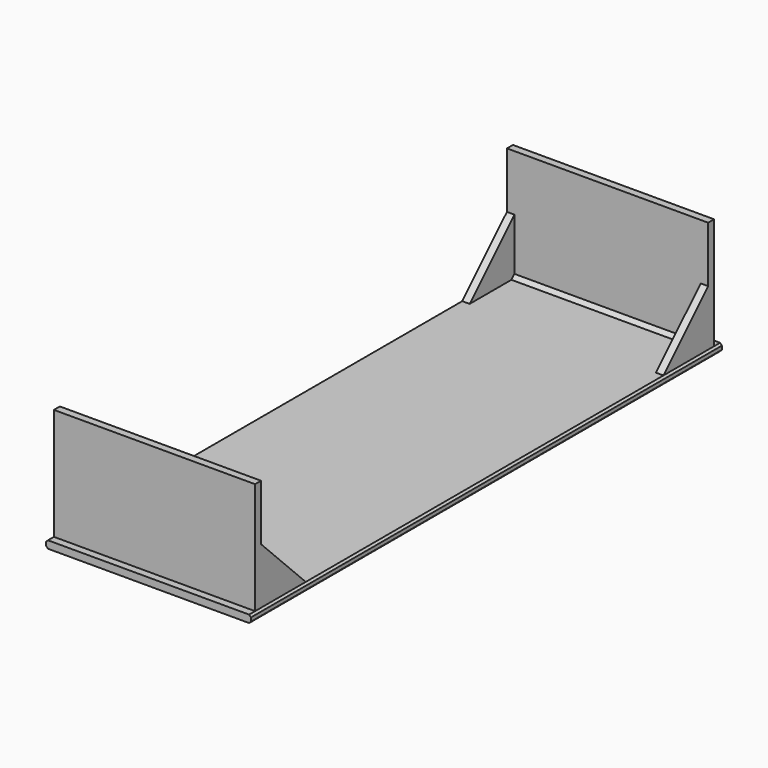
from build123d import *

# Parameters (mm, degrees)
F4_DEPTH = 27.5
F5_DEPTH = 27
F6_DEPTH = 25
F7_SIZE  = 1
F8_SIZE  = 0.49999


# Not quite as in the source:
# - a fillet or chamfer is up to 0.001 mm smaller than in the source, because OpenCascade refuses the exact size


with BuildPart() as f4:
    # F3 (on Right) → F4 (new body, symmetric)
    with BuildSketch(Plane.YZ):
        Polygon((-75, 2), (-77, 2), (-79, 2), (-79, 0), (-77, 0), (0, 0), (77, 0), (79, 0), (79, 2), (77, 2), (75, 2), (60, 2), (0, 2), (-60, 2), align=None)
    extrude(amount=F4_DEPTH, both=True)

    # F3 (on Right) → F5 (join, symmetric)
    with BuildSketch(Plane.YZ):
        Polygon((-75, 32), (-77, 32), (-77, 2), (-75, 2), (-75, 17), align=None)
        Polygon((75, 32), (75, 17), (75, 2), (77, 2), (77, 32), align=None)
        Polygon((-75, 17), (-75, 2), (-60, 2), align=None)
        Polygon((75, 17), (60, 2), (75, 2), align=None)
    extrude(amount=F5_DEPTH, both=True)

    # F3 (on Right) → F6 (cut, symmetric)
    with BuildSketch(Plane.YZ):
        Polygon((-75, 17), (-75, 2), (-60, 2), align=None)
        Polygon((75, 17), (60, 2), (75, 2), align=None)
    extrude(amount=F6_DEPTH, both=True, mode=Mode.SUBTRACT)

    # F7
    f7_edges = [f4.edges().sort_by_distance(p)[0] for p in [
        (0, -75, 2),
        (0, 75, 2),
    ]]
    chamfer(f7_edges, length=F7_SIZE)

    # F8 (size 0.5 in the source; OpenCascade refuses exactly that, so slightly less here)
    f8_edges = [f4.edges().sort_by_distance(p)[0] for p in [
        (27.5, 0, 2),
        (27.5, 0, 0),
        (-27.5, 0, 2),
        (-27.5, 0, 0),
    ]]
    chamfer(f8_edges, length=F8_SIZE)


solid = f4.part
